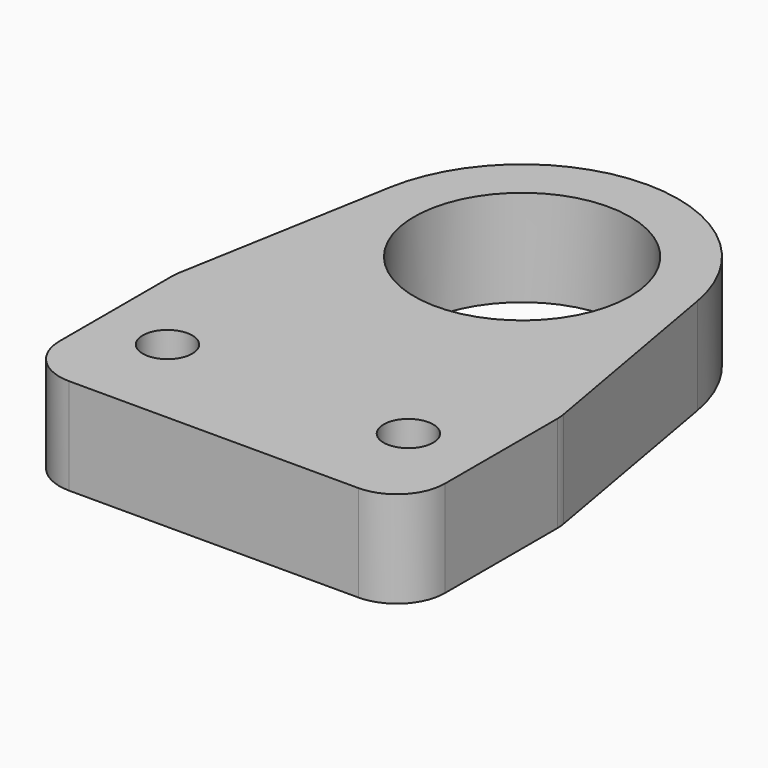
from build123d import *

# Parameters (mm, degrees)
F0_R     = 3.2639
F0_R_2   = 14.224
F1_DEPTH = 12.7
F2_R     = 6.35


# Not quite as in the source:
# - ends of sketch curves that miss each other by under 0.0002 mm in the source are joined


with BuildPart() as f1:
    # F0 (on Top) → F1 (new body)
    with BuildSketch(Plane.XY):
        with BuildLine():
            Line((-19.0499999385, -12.7), (19.0500000615, -12.7))
            ThreePointArc((19.0500000615, -12.7), (23.5401281437, -10.8401280388), (25.4000000615, -6.3499999385))
            Line((25.4000000615, -6.3499999385), (25.3999998771, 12.7))
            Line((25.3999998771, 12.7), (20.257849715, 41.692909813))
            ThreePointArc((20.257849715, 41.692909813), (0, 58.674), (-20.257849715, 41.692909813))
            Line((-20.257849715, 41.692909813), (-25.4000001229, 12.7))
            Line((-25.4000001229, 12.7), (-25.3999999385, -6.3500000615))
            ThreePointArc((-25.3999999385, -6.3500000615), (-23.5401279774, -10.8401280823), (-19.0499999385, -12.7))
        make_face()
        with Locations((-16.256, 0)):
            Circle(F0_R, mode=Mode.SUBTRACT)
        with Locations((15.494, 0)):
            Circle(F0_R, mode=Mode.SUBTRACT)
        with Locations((0, 38.1)):
            Circle(F0_R_2, mode=Mode.SUBTRACT)
    extrude(amount=F1_DEPTH)

    # F2
    f2_edges = [f1.edges().sort_by_distance(p)[0] for p in [
        (25.4, 12.7, 6.35),
        (-25.4, 12.7, 6.35),
    ]]
    fillet(f2_edges, radius=F2_R)


solid = f1.part
